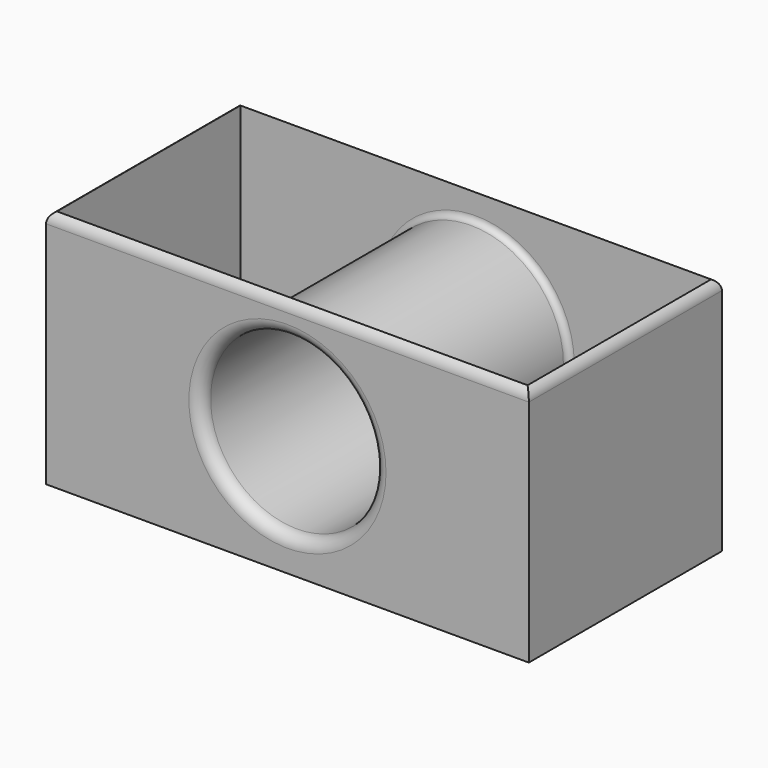
from build123d import *

# Parameters (mm, degrees)
F0_W        = 200
F0_H        = 100
F1_DEPTH    = 100
F2_R        = 35.8409251955
F3_DEPTH    = 100.001
F4_R        = 5
F5_T        = -2.5
F6_T1_DEPTH = 225
F6_T3_DEPTH = 125


# Not quite as in the source:
# - a fillet or chamfer that OpenCascade refuses, or shapes differently, is made with other operations: its cross-section is extruded or revolved along the edge and cut away or added


with BuildPart() as f1:
    # F0 (on Front) → F1 (new body)
    with BuildSketch(Plane.XZ):
        Rectangle(F0_W, F0_H)
    extrude(amount=F1_DEPTH)

    # F2 (on face) → F3 (cut, through all)
    with BuildSketch(Plane.XZ.offset(100)):
        Circle(F2_R)
    extrude(amount=-F3_DEPTH, mode=Mode.SUBTRACT)

    # F4
    f4_edges = [f1.edges().sort_by_distance(p)[0] for p in [
        (-35.840925, -100, 0),
        (-35.840925, 0, 0),
    ]]
    fillet(f4_edges, radius=F4_R)

    # F5
    f5_openings = [f1.faces().sort_by_distance(p)[0] for p in [
        (0, -50, 50),
    ]]
    offset(amount=F5_T, openings=f5_openings)

    # F6: fillet of radius 5 on 4 edges, made by hand

    # F6_s2 → F6_t1 (cut)
    with BuildSketch(Plane.YZ.offset(-112.5)):
        with BuildLine():
            ThreePointArc((-100, 45), (-98.5355339059, 48.5355339059), (-95, 50))
            Line((-95, 50), (-100, 50))
            Line((-100, 50), (-100, 45))
        make_face()
        with BuildLine():
            ThreePointArc((0, 45), (-1.4644660941, 48.5355339059), (-5, 50))
            Line((-5, 50), (0, 50))
            Line((0, 50), (0, 45))
        make_face()
    extrude(amount=F6_T1_DEPTH, mode=Mode.SUBTRACT)

    # F6_s4 → F6_t3 (cut)
    with BuildSketch(Plane.XZ.offset(-12.5)):
        with BuildLine():
            ThreePointArc((-100, 45), (-98.5355339059, 48.5355339059), (-95, 50))
            Line((-95, 50), (-100, 50))
            Line((-100, 50), (-100, 45))
        make_face()
        with BuildLine():
            ThreePointArc((100, 45), (98.5355339059, 48.5355339059), (95, 50))
            Line((95, 50), (100, 50))
            Line((100, 50), (100, 45))
        make_face()
    extrude(amount=F6_T3_DEPTH, mode=Mode.SUBTRACT)


solid = f1.part
